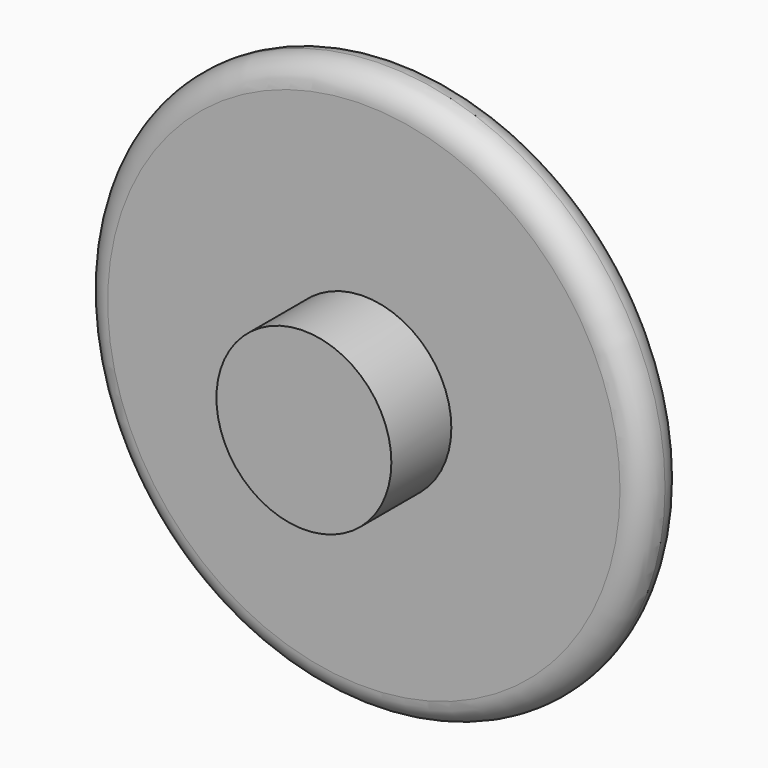
from build123d import *

# Parameters (mm, degrees)
F0_R     = 3.5
F1_DEPTH = 5
F0_R_2   = 11.25
F2_DEPTH = 2
F3_R     = 0.99999


# Not quite as in the source:
# - a fillet or chamfer is up to 0.001 mm smaller than in the source, because OpenCascade refuses the exact size


with BuildPart() as f1:
    # F0 (on Front) → F1 (new body)
    with BuildSketch(Plane.XZ):
        Circle(F0_R)
    extrude(amount=F1_DEPTH)

    # F0 (on Front) → F2 (join)
    with BuildSketch(Plane.XZ):
        Circle(F0_R_2)
        Circle(F0_R, mode=Mode.SUBTRACT)
    extrude(amount=F2_DEPTH)

    # F3 (radius 1 in the source; OpenCascade refuses exactly that, so slightly less here)
    f3_edges = [f1.edges().sort_by_distance(p)[0] for p in [
        (-11.25, -2, 0),
        (-11.25, 0, 0),
    ]]
    fillet(f3_edges, radius=F3_R)


solid = f1.part
